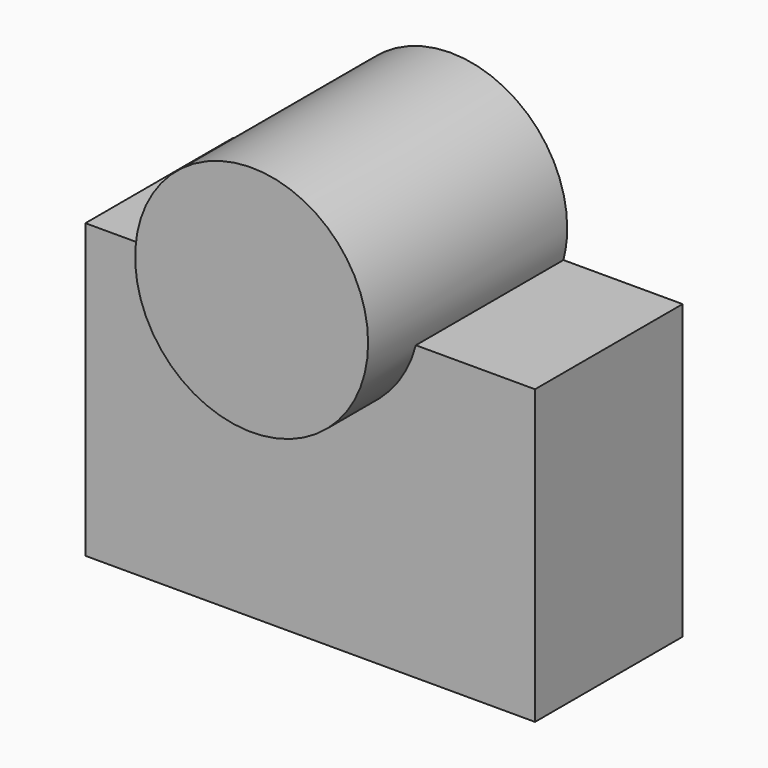
from build123d import *

# Parameters (mm, degrees)
F0_W     = 118.8637800515
F0_H     = 77.4197466671
F1_DEPTH = 48.768
F4_R     = 30.7965572654
F5_DEPTH = 65.786


# Not quite as in the source:
# - the program builds the solid bodies; features that only make, move or delete a surface that nothing else refers to are left out


with BuildPart() as f1:
    # F0 (on Front) → F1 (new body)
    with BuildSketch(Plane.XZ):
        with Locations((1.8707383424, -0.1439023763)):
            Rectangle(F0_W, F0_H)
    extrude(amount=F1_DEPTH)

    # F4 (on Front) → F5 (join)
    with BuildSketch(Plane.XZ):
        with Locations((0, 46.3367253542)):
            Circle(F4_R)
    extrude(amount=F5_DEPTH)


solid = f1.part
